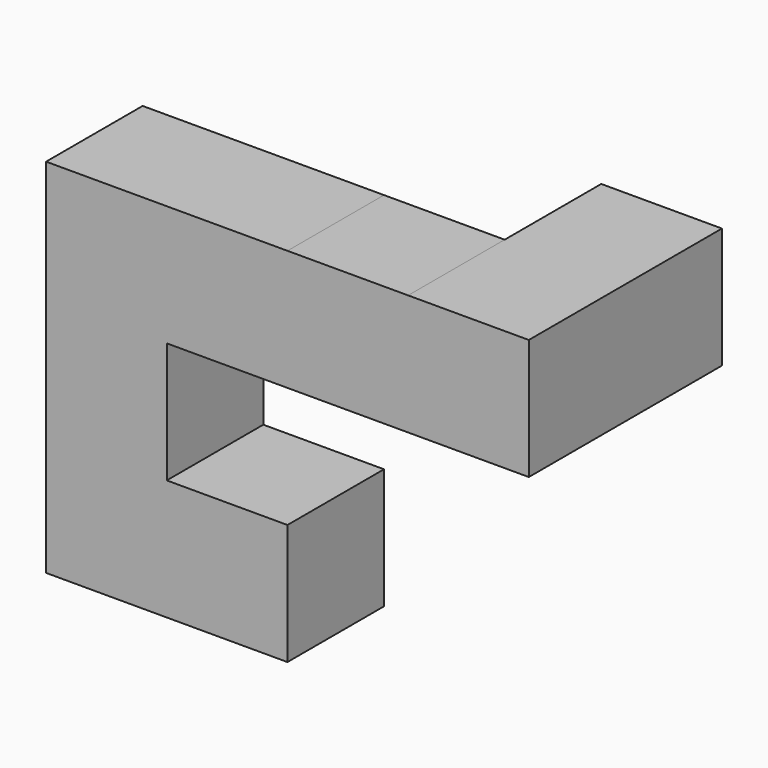
from build123d import *

# Parameters (mm, degrees)
F1_DEPTH = 12.7
F0_W     = 12.7
F0_H     = 12.7
F2_DEPTH = 12.7


# Not quite as in the source:
# - ends of sketch curves that miss each other by under 0.0002 mm in the source are joined


with BuildPart() as f1:
    # F0 (on Front) → F1 (new body, symmetric)
    with BuildSketch(Plane.XZ):
        Polygon((-29.5039405265, 55.3395837995), (-29.5039405265, 42.6395821044), (-16.8039405265, 42.6395821044), (-16.8039405265, 55.3395821044), align=None)
    extrude(amount=F1_DEPTH, both=True)

    # F0 (on Front) → F2 (join)
    with BuildSketch(Plane.XZ):
        Polygon((-42.2039422216, 55.3395821044), (-42.2039422216, 42.6395821044), (-29.5039405265, 42.6395821044), (-29.5039405265, 55.3395837995), align=None)
        with Locations((-48.5539422216, 48.9895821044)):
            Rectangle(F0_W, F0_H)
        with Locations((-61.2539422216, 48.9895821044)):
            Rectangle(F0_W, F0_H)
        with Locations((-61.2539422216, 36.2895821044)):
            Rectangle(F0_W, F0_H)
        with Locations((-61.2539422216, 23.5895821044)):
            Rectangle(F0_W, F0_H)
        with Locations((-48.5539422216, 23.5895821044)):
            Rectangle(F0_W, F0_H)
    extrude(amount=F2_DEPTH)


solid = f1.part
